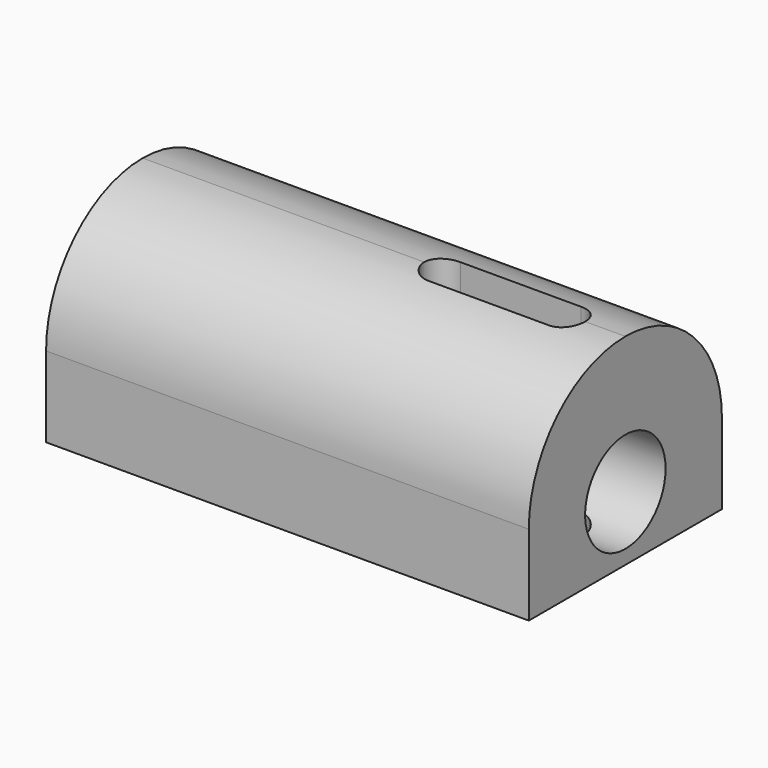
from build123d import *

# Parameters (mm, degrees)
F0_W     = 12
F0_H     = 6
F1_DEPTH = 5
F2_R     = 2.99999
F3_R     = 1.25
F4_DEPTH = 25
F6_DEPTH = 25


# Not quite as in the source:
# - a fillet or chamfer is up to 0.001 mm smaller than in the source, because OpenCascade refuses the exact size


with BuildPart() as f1:
    # F0 (on Top) → F1 (new body)
    with BuildSketch(Plane.XY):
        with Locations((12.4557307512, 0)):
            Rectangle(F0_W, F0_H)
    extrude(amount=F1_DEPTH)

    # F2 (radius 3 in the source; OpenCascade refuses exactly that, so slightly less here)
    f2_edges = [f1.edges().sort_by_distance(p)[0] for p in [
        (12.455731, -3, 5),
        (12.455731, 3, 5),
    ]]
    fillet(f2_edges, radius=F2_R)

    # F3 (on face) → F4 (cut)
    with BuildSketch(Plane.YZ.offset(18.4557307512)):
        with Locations((0, 1.6)):
            Circle(F3_R)
    extrude(amount=-F4_DEPTH, mode=Mode.SUBTRACT)

    # F5 (on face) → F6 (cut)
    with BuildSketch(Plane(origin=(0, 0, 0), x_dir=(1, 0, 0), z_dir=(0, 0, -1))):
        with BuildLine():
            Line((13.9557307512, -0.5), (16.9557307512, -0.5))
            ThreePointArc((16.9557307512, -0.5), (17.4557307512, 0), (16.9557307512, 0.5))
            Line((16.9557307512, 0.5), (13.9557307512, 0.5))
            ThreePointArc((13.9557307512, 0.5), (13.4557307512, 0), (13.9557307512, -0.5))
        make_face()
    extrude(amount=-F6_DEPTH, mode=Mode.SUBTRACT)


solid = f1.part
